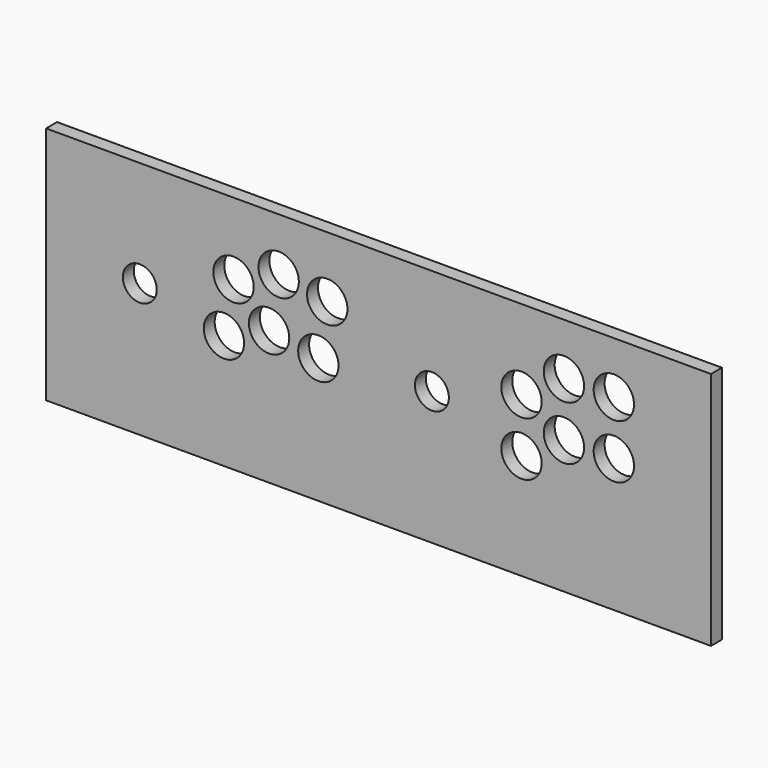
from build123d import *

# Parameters (mm, degrees)
F0_W     = 486
F0_H     = 175
F1_DEPTH = 10
F5_R     = 14.75
F5_R_2   = 12.4064380464
F7_DEPTH = 25
F3_R     = 14.75
F3_R_2   = 12.4065
F8_DEPTH = 25


# Not quite as in the source:
# - a feature names something its author has since deleted; it is built from what else it names


with BuildPart() as f1:
    # F0 (on Front) → F1 (new body)
    with BuildSketch(Plane.XZ):
        with Locations((243, 87.5)):
            Rectangle(F0_W, F0_H)
    extrude(amount=F1_DEPTH)

    # F5 (on face) → F7 (cut)
    with BuildSketch(Plane.XZ.offset(10)):
        with Locations((347.5, 116.75)):
            Circle(F5_R)
        with Locations((378.5, 137)):
            Circle(F5_R)
        with Locations((415, 137)):
            Circle(F5_R)
        with Locations((415, 97.5)):
            Circle(F5_R)
        with Locations((378.5, 97.5)):
            Circle(F5_R)
        with Locations((347.5, 77.25)):
            Circle(F5_R)
        with Locations((282, 97.5)):
            Circle(F5_R_2)
    extrude(amount=-F7_DEPTH, mode=Mode.SUBTRACT)

    # F3 (on face) → F8 (cut)
    with BuildSketch(Plane.XZ.offset(10)):
        with Locations((170, 136.3350188136)):
            Circle(F3_R)
        with Locations((205.5, 130.3350188136)):
            Circle(F3_R)
        with Locations((199, 91.8350188136)):
            Circle(F3_R)
        with Locations((163, 97.8350188136)):
            Circle(F3_R)
        with Locations((130, 83.8350188136)):
            Circle(F3_R)
        with Locations((137, 122.3350188136)):
            Circle(F3_R)
        with Locations((68.5, 97.5)):
            Circle(F3_R_2)
    extrude(amount=-F8_DEPTH, mode=Mode.SUBTRACT)


solid = f1.part
